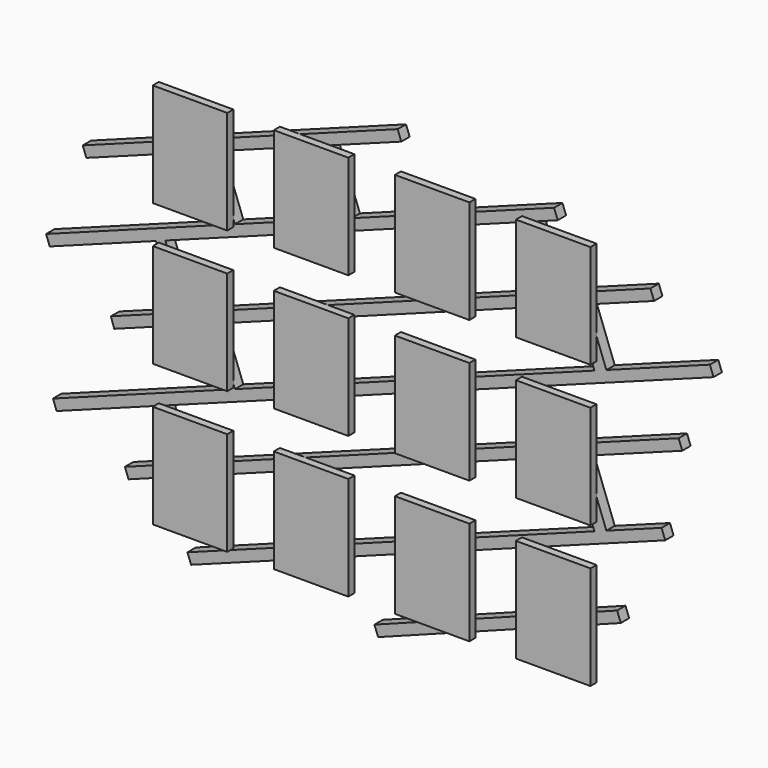
from build123d import *

# Parameters (mm, degrees)
F0_W     = 128
F0_H     = 178
F1_DEPTH = 13
F3_DEPTH = 18


# Not quite as in the source:
# - a feature names something its author has since deleted; it is built from what else it names


with BuildPart() as f1:
    # F0 (on Front) → F1 (new body)
    with BuildSketch(Plane.XZ):
        with Locations((219.08757779, -59.0834027313)):
            Rectangle(F0_W, F0_H)
    extrude(amount=F1_DEPTH)


with BuildPart() as f1b:
    # F0 (on Front) → F1, piece 2 (new body)
    with BuildSketch(Plane.XZ):
        with Locations((11.08757779, -59.0834027313)):
            Rectangle(F0_W, F0_H)
    extrude(amount=F1_DEPTH)


with BuildPart() as f1c:
    # F0 (on Front) → F1, piece 3 (new body)
    with BuildSketch(Plane.XZ):
        with Locations((427.08757779, -59.0834027313)):
            Rectangle(F0_W, F0_H)
    extrude(amount=F1_DEPTH)


with BuildPart() as f1d:
    # F0 (on Front) → F1, piece 4 (new body)
    with BuildSketch(Plane.XZ):
        with Locations((635.08757779, -545.0834027313)):
            Rectangle(F0_W, F0_H)
    extrude(amount=F1_DEPTH)


with BuildPart() as f1e:
    # F0 (on Front) → F1, piece 5 (new body)
    with BuildSketch(Plane.XZ):
        with Locations((635.08757779, -59.0834027313)):
            Rectangle(F0_W, F0_H)
    extrude(amount=F1_DEPTH)


with BuildPart() as f1f:
    # F0 (on Front) → F1, piece 6 (new body)
    with BuildSketch(Plane.XZ):
        with Locations((427.08757779, -302.0834027313)):
            Rectangle(F0_W, F0_H)
    extrude(amount=F1_DEPTH)


with BuildPart() as f1g:
    # F0 (on Front) → F1, piece 7 (new body)
    with BuildSketch(Plane.XZ):
        with Locations((11.08757779, -302.0834027313)):
            Rectangle(F0_W, F0_H)
    extrude(amount=F1_DEPTH)


with BuildPart() as f1h:
    # F0 (on Front) → F1, piece 8 (new body)
    with BuildSketch(Plane.XZ):
        with Locations((219.08757779, -545.0834027313)):
            Rectangle(F0_W, F0_H)
    extrude(amount=F1_DEPTH)


with BuildPart() as f1i:
    # F0 (on Front) → F1, piece 9 (new body)
    with BuildSketch(Plane.XZ):
        with Locations((427.08757779, -545.0834027313)):
            Rectangle(F0_W, F0_H)
    extrude(amount=F1_DEPTH)


with BuildPart() as f1j:
    # F0 (on Front) → F1, piece 10 (new body)
    with BuildSketch(Plane.XZ):
        with Locations((219.08757779, -302.0834027313)):
            Rectangle(F0_W, F0_H)
    extrude(amount=F1_DEPTH)


with BuildPart() as f1k:
    # F0 (on Front) → F1, piece 11 (new body)
    with BuildSketch(Plane.XZ):
        with Locations((11.08757779, -545.0834027313)):
            Rectangle(F0_W, F0_H)
    extrude(amount=F1_DEPTH)


with BuildPart() as f1l:
    # F0 (on Front) → F1, piece 12 (new body)
    with BuildSketch(Plane.XZ):
        with Locations((635.08757779, -302.0834027313)):
            Rectangle(F0_W, F0_H)
    extrude(amount=F1_DEPTH)


with BuildPart() as f3:
    # F2 (on Front) → F3 (new body)
    with BuildSketch(Plane.XZ):
        Polygon((60.4232248307, -398.7421964755), (-234.7520887852, -508.1428327886), (-228.4965866558, -525.0208863822), (-57.9250411064, -461.8020643492), (-28.7042035388, -540.6431952952), (-111.1862889092, -571.2134774553), (-104.9307867798, -588.091531049), (168.0806095152, -486.905493133), (205.552702723, -588.0094467955), (-3.7035272283, -665.565948485), (2.5519749011, -682.4440020786), (393.5769142789, -537.5186807223), (427.5221156744, -629.1066806219), (317.5466656685, -670.4911589622), (323.886180298, -687.3378368028), (740.8686522409, -530.4246159204), (734.5291376114, -513.5779380798), (638.1482213573, -549.8467047994), (604.1415982984, -459.4772275445), (817.192169836, -380.5144314774), (810.9366677066, -363.6363778838), (716.0965861902, -398.7868961937), (678.6244929824, -297.6829425311), (846.5011555757, -235.4629232319), (840.2456534463, -218.5848696383), (631.5366836103, -295.9385406639), (602.3158460427, -217.0974097179), (900.2279571147, -106.6824359269), (893.9724549853, -89.8043823333), (716.0965861902, -155.7304009849), (683.2807828027, -67.1896448896), (798.0482913025, -24.6534371555), (791.7927891732, -7.7753835618), (631.5366836103, -67.1710007186), (595.5626142285, 29.8911149113), (632.4966396134, 43.5799489443), (626.241137484, 60.4580025379), (278.2693529878, -68.5105557624), (241.7988051832, 29.8911149113), (363.7198763254, 75.0786429588), (357.464374196, 91.9566965524), (-183.6906183795, -108.6112296964), (-177.4351162501, -125.48928329), (24.3737957177, -50.6929762666), (60.8443435224, -149.0946469404), (-246.5978554338, -263.041751064), (-240.3423533044, -279.9198046577), (-57.9250411064, -212.3105937635), (-22.5504447533, -309.5948916958), (-135.233659056, -351.3585988145), (-129.5387379368, -368.4444201868), (27.6074214432, -310.2014403802), align=None)
        Polygon((582.3585393656, -224.4941734338), (611.5793769332, -303.3353043797), (-12.4146006773, -534.6057902815), (-41.6354382449, -455.7646593355), align=None, mode=Mode.SUBTRACT)
        Polygon((443.7871834658, -622.9860296432), (409.8720723686, -531.479216778), (586.8097008915, -465.900937514), (620.8487580962, -556.3566055326), align=None, mode=Mode.SUBTRACT)
        Polygon((184.9646659648, -480.6477661689), (658.1168387539, -305.2836812054), (695.5889319617, -406.3876348679), (222.4367591726, -581.7517198314), align=None, mode=Mode.SUBTRACT)
        Polygon((575.1038426377, 22.3084935776), (611.0779120195, -74.7536220523), (-5.6613688631, -303.3353043797), (-41.6354382449, -206.2731887499), align=None, mode=Mode.SUBTRACT)
        Polygon((77.8530937728, -142.7907047933), (41.3825459681, -44.3890341195), (220.9827505318, 22.176073987), (257.4532983364, -76.2255966867), align=None, mode=Mode.SUBTRACT)
        Polygon((45.0372903853, -303.7414192837), (662.872315298, -74.7536220523), (695.6881186856, -163.2943781476), (77.8530937728, -392.282175379), align=None, mode=Mode.SUBTRACT)
    extrude(amount=-F3_DEPTH)


solid = Compound([f1.part, f1b.part, f1c.part, f1d.part, f1e.part, f1f.part, f1g.part, f1h.part, f1i.part, f1j.part, f1k.part, f1l.part, f3.part])
